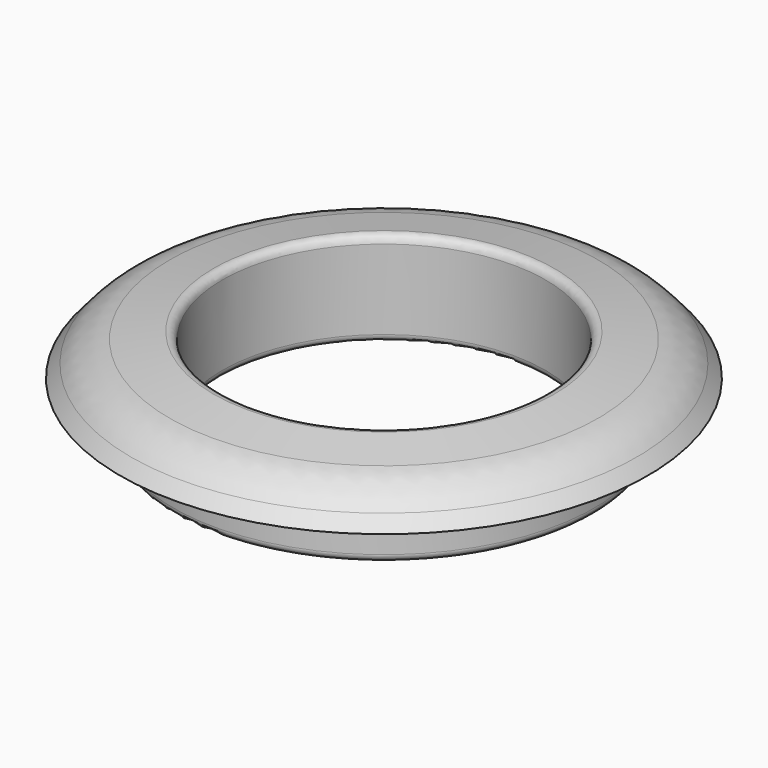
from build123d import *

# Parameters (mm, degrees)
F3_R = 7.62
F4_R = 0.889


# Not quite as in the source:
# - a fillet or chamfer that OpenCascade refuses, or shapes differently, is made with other operations: its cross-section is extruded or revolved along the edge and cut away or added


with BuildPart() as f1:
    # F0 (on Front) → F1 (revolve)
    with BuildSketch(Plane.XZ):
        Polygon((-25.146, 6.35), (-25.146, 0), (-19.304, 0), (-19.304, 11.43), (-31.496, 9.525), (-31.496, 6.35), align=None)
    revolve(axis=Axis((0, 0, 48.3202852037), (0, 0, 1)))

    # F2: chamfer of 3.175 on 1 edges, made by hand

    # F2_s1 → F2_t2 (revolve, cut)
    with BuildSketch(Plane.XZ):
        Polygon((-28.3590617928, 10.0151465949), (-31.496, 6.35), (-31.496, 9.525), align=None)
    revolve(axis=Axis((0, 0, 9.525), (0, 0, 1)), mode=Mode.SUBTRACT)

    # F3
    f3_edges = [f1.edges().sort_by_distance(p)[0] for p in [
        (28.359062, 0, 10.015147),
    ]]
    fillet(f3_edges, radius=F3_R)

    # F4
    f4_edges = [f1.edges().sort_by_distance(p)[0] for p in [
        (19.304, 0, 11.43),
        (19.304, 0, 0),
        (25.146, 0, 0),
    ]]
    fillet(f4_edges, radius=F4_R)


solid = f1.part
